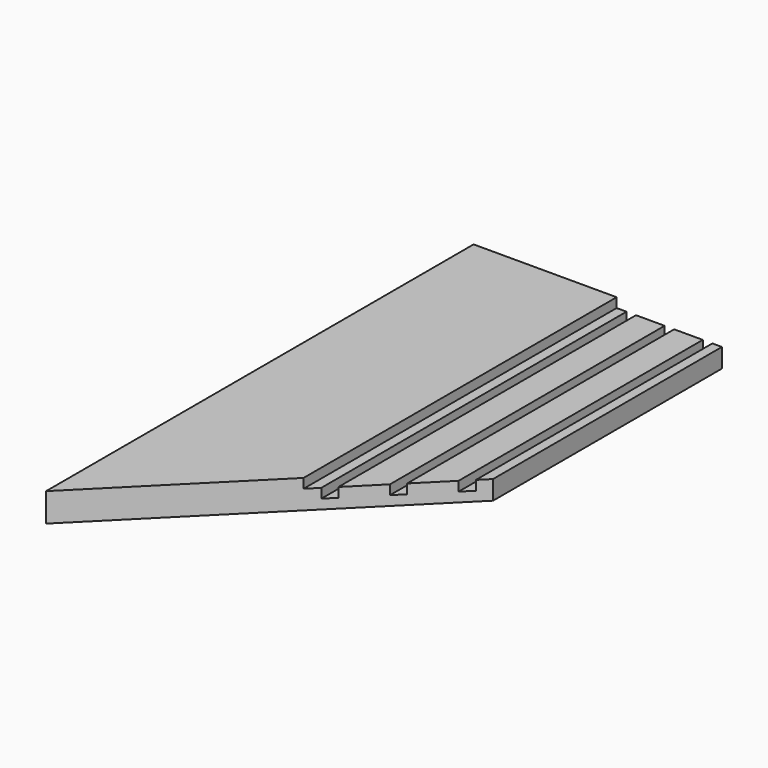
from build123d import *

# Parameters (mm, degrees)
F0_W        = 30
F0_H        = 10
F0_W_2      = 10.3326633751
F1_DEPTH    = 300
F2_T1_DEPTH = 1563.0097927795


# Not quite as in the source:
# - a fillet or chamfer that OpenCascade refuses, or shapes differently, is made with other operations: its cross-section is extruded or revolved along the edge and cut away or added


with BuildPart() as f1:
    # F0 (on Front) → F1 (new body, symmetric)
    with BuildSketch(Plane.XZ):
        Polygon((-41.8675842226, -17.4409984683), (-41.8675842226, -7.4409984683), (-191.8675842226, -7.4409984683), (-191.8675842226, -37.4409984683), (-41.8675842226, -37.4409984683), (-41.8675842226, -27.4409984683), align=None)
        with Locations((33.4650791525, -22.4409984683)):
            Rectangle(F0_W, F0_H)
        with Locations((-36.7012525351, -22.4409984683)):
            Rectangle(F0_W_2, F0_H)
        with Locations((-6.5349208475, -22.4409984683)):
            Rectangle(F0_W, F0_H)
        Polygon((-31.5349208475, -27.4409984683), (-41.8675842226, -27.4409984683), (-41.8675842226, -37.4409984683), (58.5501386541, -37.4409984683), (58.5501386541, -27.4409984683), (48.4650791525, -27.4409984683), (18.4650791525, -27.4409984683), (8.4650791525, -27.4409984683), (-21.5349208475, -27.4409984683), align=None)
        Polygon((58.5501386541, -27.4409984683), (58.5501386541, -37.4409984683), (68.5501386541, -37.4409984683), (68.5501386541, -17.4409984683), (58.5501386541, -17.4409984683), align=None)
    extrude(amount=F1_DEPTH, both=True)

    # F2: chamfer of 300 on 1 edges, made by hand

    # F2_s2 → F2_t1 (cut)
    with BuildSketch(Plane.XY.offset(-808.945894858)):
        Polygon((68.5501386541, 0), (-231.4498613459, -300), (68.5501386541, -300), align=None)
    extrude(amount=F2_T1_DEPTH, mode=Mode.SUBTRACT)


solid = f1.part
